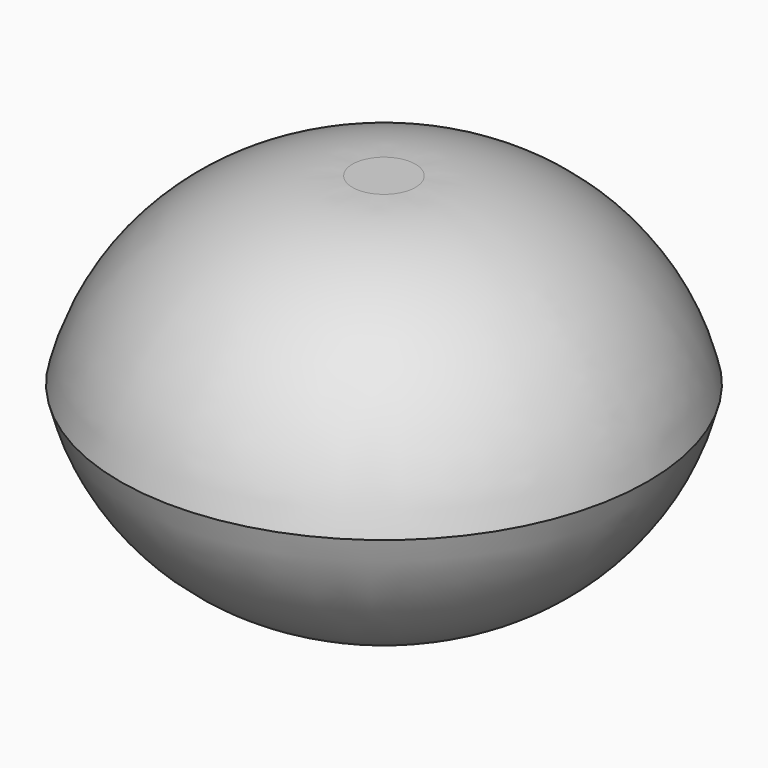
from build123d import *

# Parameters (mm, degrees)
F0_R     = 36.5668122635
F1_DEPTH = 25.4


# Not quite as in the source:
# - a fillet or chamfer that OpenCascade refuses, or shapes differently, is made with other operations: its cross-section is extruded or revolved along the edge and cut away or added


with BuildPart() as f1:
    # F0 (on Top) → F1 (new body)
    with BuildSketch(Plane.XY):
        Circle(F0_R)
    extrude(amount=F1_DEPTH)

    # F2: fillet of radius 33.1133532215 on 1 edges, made by hand

    # F2_s1 → F2_t2 (revolve, cut)
    with BuildSketch(Plane.XZ):
        with BuildLine():
            ThreePointArc((36.5668122635, 0), (24.8714154597, 18.2857732188), (4.364353605, 25.4))
            Line((4.364353605, 25.4), (36.5668122635, 25.4))
            Line((36.5668122635, 25.4), (36.5668122635, 0))
        make_face()
    revolve(axis=Axis((0, 0, 25.4), (0, 0, 1)), mode=Mode.SUBTRACT)

    # F3: F1 across plane


with BuildPart() as f1_1:
    add(f1.part)
    add(f1.part.mirror(Plane.XY))


solid = f1_1.part
